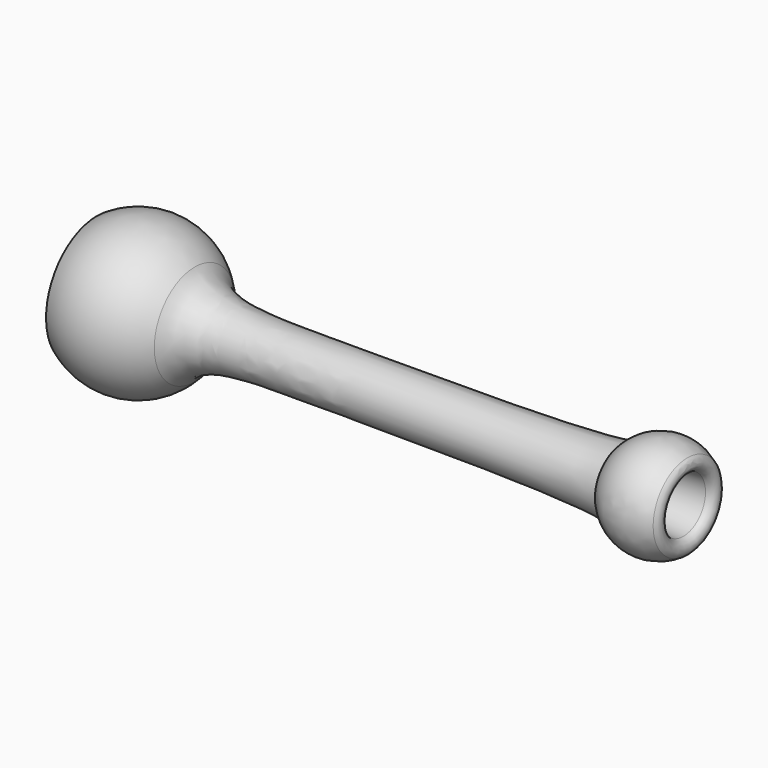
from build123d import *

# Parameters (mm, degrees)
F2_R = 2


# Not quite as in the source:
# - a fillet or chamfer that OpenCascade refuses, or shapes differently, is made with other operations: its cross-section is extruded or revolved along the edge and cut away or added


with BuildPart() as f1:
    # F0 (on Front) → F1 (revolve)
    with BuildSketch(Plane.XZ):
        with BuildLine():
            ThreePointArc((-7.0685046336, 10.3095219212), (4.6853520259, 11.5886788028), (12.2474487139, 2.5))
            Line((12.2474487139, 2.5), (74.2474487139, 2.5))
            Line((74.2474487139, 2.5), (137.0374359825, 7.0690793239))
            ThreePointArc((137.0374359825, 7.0690793239), (127.7669650478, 12.4694859534), (117.8826543599, 8.2973851228))
            add(Edge.make_bspline(
                [(13.7809895682, 12.3177978136), (17.3247616462, 6.4736620698), (43.5822553755, 6.750698096), (109.6914496017, 6.3752606308), (117.8826543599, 8.2973851228)],
                knots=[0, 0, 0, 0, 0.3926023717, 1, 1, 1, 1], degree=3))
            ThreePointArc((13.7809895682, 12.3177978136), (2.4835532955, 18.3159979112), (-10.003236638, 15.5428141988))
            Line((-10.003236638, 15.5428141988), (-7.0685046336, 10.3095219212))
        make_face()
    revolve(axis=Axis((35, 0, 0), (1, 0, 0)))

    # F2
    f2_edges = [f1.edges().sort_by_distance(p)[0] for p in [
        (137.037436, 0, -7.069079),
        (-7.068505, 0, -10.309522),
        (12.247449, 0, -2.5),
    ]]
    fillet(f2_edges, radius=F2_R)

    # F3: fillet of radius 5 on 1 edges, made by hand

    # F3_s1 → F3_t2 (revolve, cut)
    with BuildSketch(Plane.XZ):
        with BuildLine():
            ThreePointArc((74.0656971228, 2.4996), (74.247343375, 2.5028990409), (74.4287500388, 2.5127918123))
            Line((74.4287500388, 2.5127918123), (74.4650553304, 2.0138709935))
            ThreePointArc((74.4650553304, 2.0138709935), (74.3743901528, 2.00767456), (74.2837540055, 2.0010791812))
            Line((74.2837540055, 2.0010791812), (74.2474487139, 1.99976))
            ThreePointArc((74.2474487139, 1.99976), (74.1565729184, 1.99976), (74.0656971228, 1.99936))
            Line((74.0656971228, 1.99936), (74.0656971228, 2.4996))
        make_face()
    revolve(axis=Axis((74.2474487139, 0, 0), (1, 0, 0)), mode=Mode.SUBTRACT)


solid = f1.part
